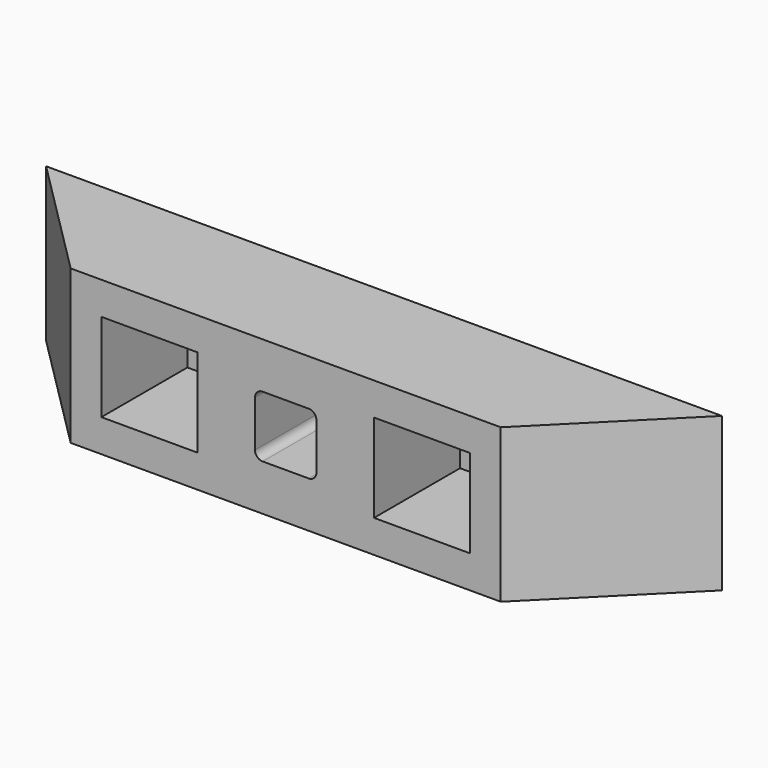
from build123d import *

# Parameters (mm, degrees)
F1_DEPTH = 127
F3_DEPTH = 101.601
F4_W     = 79.375
F4_H     = 36.5125
F5_DEPTH = 88.9


# Not quite as in the source:
# - a feature names something its author has since deleted; it is built from what else it names


with BuildPart() as f1:
    # F0 (on Top) → F1 (new body)
    with BuildSketch(Plane.XY):
        Polygon((177.8, 0), (-177.8, 0), (-279.4, 0), (-177.8, -101.6), (177.8, -101.6), (279.4, 0), align=None)
    extrude(amount=F1_DEPTH)

    # F2 (on face) → F3 (cut, through all)
    with BuildSketch(Plane.XZ.offset(101.6)):
        with BuildLine():
            Line((19.05, 88.9), (-19.05, 88.9))
            ThreePointArc((-19.05, 88.9), (-23.5401280605, 87.0401280605), (-25.4, 82.55))
            Line((-25.4, 82.55), (-25.4, 44.45))
            ThreePointArc((-25.4, 44.45), (-23.5401280605, 39.9598719395), (-19.05, 38.1))
            Line((-19.05, 38.1), (19.05, 38.1))
            ThreePointArc((19.05, 38.1), (23.5401280605, 39.9598719395), (25.4, 44.45))
            Line((25.4, 44.45), (25.4, 82.55))
            ThreePointArc((25.4, 82.55), (23.5401280605, 87.0401280605), (19.05, 88.9))
        make_face()
    extrude(amount=-F3_DEPTH, mode=Mode.SUBTRACT)

    # F4 (on face) → F5 (cut)
    with BuildSketch(Plane.XZ.offset(101.6)):
        with Locations((-112.7125, 45.24375)):
            Rectangle(F4_W, F4_H)
        with Locations((-112.7125, 81.75625)):
            Rectangle(F4_W, F4_H)
        with Locations((112.7125, 81.75625)):
            Rectangle(F4_W, F4_H)
        with Locations((112.7125, 45.24375)):
            Rectangle(F4_W, F4_H)
    extrude(amount=-F5_DEPTH, mode=Mode.SUBTRACT)


solid = f1.part
